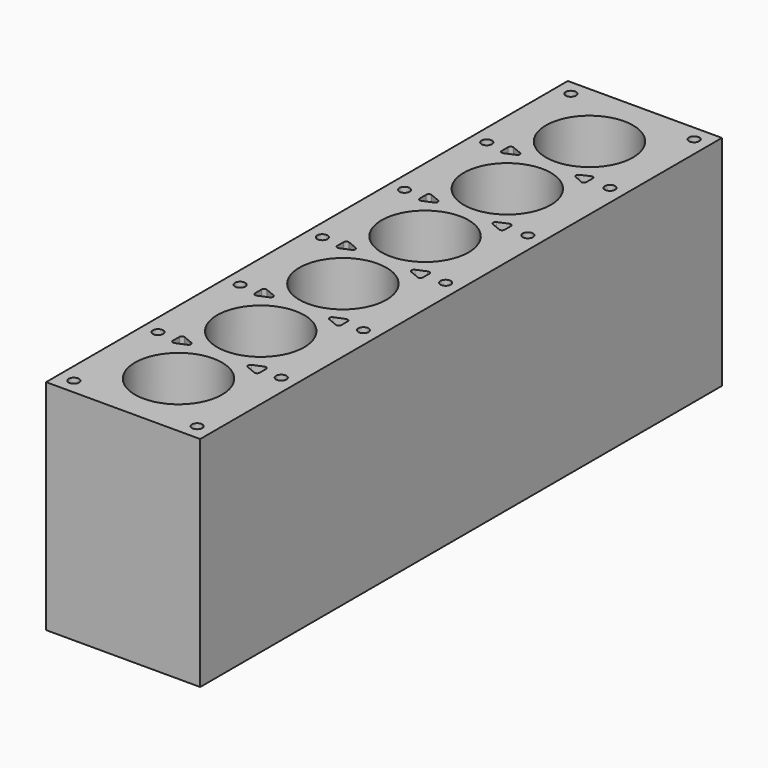
from build123d import *

# Parameters (mm, degrees)
F0_W     = 152.4
F0_H     = 644.906
F0_R     = 43.053
F1_DEPTH = 177.8
F3_D     = 10.16
F3_DEPTH = 50.8
F3_TIP   = 3.0523719447
F5_DEPTH = 101.6
F8_DEPTH = 38.1
F9_D     = 6.35
F9_DEPTH = 38.1
F9_TIP   = 1.9077324654
F10_R    = 6.35


# Not quite as in the source:
# - a feature names something its author has since deleted; it is built from what else it names


with BuildPart() as f1:
    # F0 (on Top) → F1 (new body)
    with BuildSketch(Plane.XY):
        with Locations((0, 22.9516405373)):
            Rectangle(F0_W, F0_H)
        with Locations((0, -231.0483594627)):
            Circle(F0_R, mode=Mode.SUBTRACT)
        with Locations((0, -129.4483594627)):
            Circle(F0_R, mode=Mode.SUBTRACT)
        with Locations((0, -27.8483594627)):
            Circle(F0_R, mode=Mode.SUBTRACT)
        with Locations((0, 73.7516405373)):
            Circle(F0_R, mode=Mode.SUBTRACT)
        with Locations((0, 175.3516405373)):
            Circle(F0_R, mode=Mode.SUBTRACT)
        with Locations((0, 276.9516405373)):
            Circle(F0_R, mode=Mode.SUBTRACT)
    extrude(amount=F1_DEPTH)

    # F3
    with Locations(Plane.XY.offset(177.8)):
        with Locations((-60.96, -284.2613594627), (60.96, -284.2613594627), (-60.96, -180.2483594627), (60.96, -180.2483594627), (-60.96, -78.6483594627), (60.96, -78.6483594627), (-60.96, 22.9516405373), (60.96, 22.9516405373), (-60.96, 124.5516405373), (60.96, 124.5516405373), (-60.96, 226.1516405373), (60.96, 226.1516405373), (-60.96, 330.1646405373), (60.96, 330.1646405373)):
            Hole(F3_D / 2, depth=F3_DEPTH)
            with Locations((0, 0, -(F3_DEPTH + F3_TIP / 2))):  # 118° drill point
                Cone(0, F3_D / 2, F3_TIP, mode=Mode.SUBTRACT)

    # F4 (on face) → F5 (cut)
    with BuildSketch(Plane.XY.offset(177.8)):
        with BuildLine():
            ThreePointArc((-39.5301250083, -173.9482047983), (-41.9112858201, -174.185525814), (-43.0385000083, -176.2963636216))
            Line((-43.0385000083, -176.2963636216), (-43.0385000083, -184.2003553039))
            ThreePointArc((-43.0385000083, -184.2003553039), (-41.9112858201, -186.3111931115), (-39.5301250083, -186.5485141272))
            Line((-39.5301250083, -186.5485141272), (-29.947149504, -182.596518286))
            ThreePointArc((-29.947149504, -182.596518286), (-28.375524504, -180.2483594627), (-29.947149504, -177.9002006395))
            Line((-29.947149504, -177.9002006395), (-39.5301250083, -173.9482047983))
        make_face()
        with BuildLine():
            Line((42.8050714591, -184.1785549312), (42.7631932188, -176.2809378323))
            ThreePointArc((42.7631932188, -176.2809378323), (41.6287769855, -174.1787422376), (39.2512218362, -173.9477486864))
            Line((39.2512218362, -173.9477486864), (29.7178532592, -177.8965572358))
            ThreePointArc((29.7178532592, -177.8965572358), (28.149861111, -180.2451799461), (29.7214853508, -182.5913737277))
            Line((29.7214853508, -182.5913737277), (39.2967321682, -186.5401822772))
            ThreePointArc((39.2967321682, -186.5401822772), (41.6834844647, -186.299108133), (42.8050714591, -184.1785549312))
        make_face()
        with BuildLine():
            ThreePointArc((-39.5301250083, -72.3482047983), (-41.9112858201, -72.585525814), (-43.0385000083, -74.6963636216))
            Line((-43.0385000083, -74.6963636216), (-43.0385000083, -82.6003553039))
            ThreePointArc((-43.0385000083, -82.6003553039), (-41.9112858201, -84.7111931115), (-39.5301250083, -84.9485141272))
            Line((-39.5301250083, -84.9485141272), (-29.947149504, -80.996518286))
            ThreePointArc((-29.947149504, -80.996518286), (-28.375524504, -78.6483594627), (-29.947149504, -76.3002006395))
            Line((-29.947149504, -76.3002006395), (-39.5301250083, -72.3482047983))
        make_face()
        with BuildLine():
            Line((42.2662900285, -82.5723412323), (42.2244772598, -74.6870711239))
            ThreePointArc((42.2244772598, -74.6870711239), (41.0880034509, -72.579426147), (38.7049289993, -72.3455539051))
            Line((38.7049289993, -72.3455539051), (29.1514032422, -76.2881889593))
            ThreePointArc((29.1514032422, -76.2881889593), (27.5756070282, -78.6451741517), (29.1550254915, -80.9997336057))
            Line((29.1550254915, -80.9997336057), (38.7503640173, -84.9423686599))
            ThreePointArc((38.7503640173, -84.9423686599), (41.1426684979, -84.6983979341), (42.2662900285, -82.5723412323))
        make_face()
        with BuildLine():
            ThreePointArc((-39.5301250083, 29.2517952017), (-41.9112858201, 29.014474186), (-43.0385000083, 26.9036363784))
            Line((-43.0385000083, 26.9036363784), (-43.0385000083, 18.9996446961))
            ThreePointArc((-43.0385000083, 18.9996446961), (-41.9112858201, 16.8888068885), (-39.5301250083, 16.6514858728))
            Line((-39.5301250083, 16.6514858728), (-29.947149504, 20.603481714))
            ThreePointArc((-29.947149504, 20.603481714), (-28.375524504, 22.9516405373), (-29.947149504, 25.2997993605))
            Line((-29.947149504, 25.2997993605), (-39.5301250083, 29.2517952017))
        make_face()
        with BuildLine():
            Line((41.7277221449, 18.9936006532), (41.6855505867, 26.946533154))
            ThreePointArc((41.6855505867, 26.946533154), (40.5605129606, 29.0230527195), (38.2087640486, 29.2396634781))
            Line((38.2087640486, 29.2396634781), (28.7869515979, 25.2631972277))
            ThreePointArc((28.7869515979, 25.2631972277), (27.2569622126, 22.9547929732), (28.7906370523, 20.6488356434))
            Line((28.7906370523, 20.6488356434), (38.2546210612, 16.672369393))
            ThreePointArc((38.2546210612, 16.672369393), (40.6154092138, 16.8989805748), (41.7277221449, 18.9936006532))
        make_face()
        with BuildLine():
            ThreePointArc((-39.2389715781, 130.8516052404), (-41.6215382557, 130.6118153154), (-42.7459306424, 128.4976098044))
            Line((-42.7459306424, 128.4976098044), (-42.7295716504, 120.5911560789))
            ThreePointArc((-42.7295716504, 120.5911560789), (-41.6001784129, 118.4841132501), (-39.2212020873, 118.2482526776))
            Line((-39.2212020873, 118.2482526776), (-29.635241547, 122.2014795403))
            ThreePointArc((-29.635241547, 122.2014795403), (-28.0636166616, 124.5504011364), (-29.6366520458, 126.8983783776))
            Line((-29.6366520458, 126.8983783776), (-39.2389715781, 130.8516052404))
        make_face()
        with BuildLine():
            Line((41.1269060209, 120.5623967021), (41.1269060209, 128.5408843724))
            ThreePointArc((41.1269060209, 128.5408843724), (40.0124074762, 130.6155991372), (37.6672454799, 130.8318480041))
            Line((37.6672454799, 130.8318480041), (28.2579874063, 126.8426041689))
            ThreePointArc((28.2579874063, 126.8426041689), (26.740926903, 124.5516405373), (28.2579874063, 122.2606769056))
            Line((28.2579874063, 122.2606769056), (37.6672454799, 118.2714330704))
            ThreePointArc((37.6672454799, 118.2714330704), (40.0124074762, 118.4876819373), (41.1269060209, 120.5623967021))
        make_face()
        with BuildLine():
            Line((-39.4786105583, 219.9656601087), (-29.866499751, 224.1805924273))
            ThreePointArc((-29.866499751, 224.1805924273), (-28.4228668084, 226.3396283374), (-29.8678000125, 228.4977942646))
            Line((-29.8678000125, 228.4977942646), (-39.5349560025, 232.4619589189))
            ThreePointArc((-39.5349560025, 232.4619589189), (-41.9134370658, 232.2213103618), (-43.0385000083, 230.1119698791))
            Line((-43.0385000083, 230.1119698791), (-43.0385000083, 222.2917467873))
            ThreePointArc((-43.0385000083, 222.2917467873), (-41.8879192273, 220.1655123145), (-39.4786105583, 219.9656601087))
        make_face()
        with BuildLine():
            Line((40.650672554, 222.1092328525), (40.6076142213, 230.2293979276))
            ThreePointArc((40.6076142213, 230.2293979276), (39.515765156, 232.1937343917), (37.2723493523, 232.3272920851))
            Line((37.2723493523, 232.3272920851), (28.7048957748, 228.2672095476))
            ThreePointArc((28.7048957748, 228.2672095476), (27.3697030623, 226.15467094), (28.7089851923, 224.0447225226))
            Line((28.7089851923, 224.0447225226), (37.3194971026, 219.9846399851))
            ThreePointArc((37.3194971026, 219.9846399851), (39.5711951198, 220.1279668388), (40.650672554, 222.1092328525))
        make_face()
    extrude(amount=-F5_DEPTH, mode=Mode.SUBTRACT)

    # F7 (on face) → F8 (join)
    with BuildSketch(Plane(origin=(0, 0, 0), x_dir=(1, 0, 0), z_dir=(0, 0, -1))):
        Polygon((76.2, -345.4046405373), (76.2, 299.4986176491), (76.2, 299.5013594627), (-76.2, 299.5013594627), (-76.2, -345.4046405373), align=None)
        Polygon((-60.96, -321.8358690433), (-60.96, 286.0599543583), (60.96, 286.0599543583), (60.96, -331.9680405373), (-60.96, -331.9680405373), align=None, mode=Mode.SUBTRACT)
    extrude(amount=F8_DEPTH)

    # F9 (one way)
    with BuildSketch(Plane.XY):
        with Locations((-68.58, -78.6483594627), (68.58, -78.6483594627)):
            Circle(F9_D / 2)
    extrude(amount=-F9_DEPTH, mode=Mode.SUBTRACT)
    with Locations(Plane.XY):
        with Locations((-68.58, -78.6483594627), (68.58, -78.6483594627)):
            with Locations((0, 0, -(F9_DEPTH + F9_TIP / 2))):  # 118° drill point
                Cone(0, F9_D / 2, F9_TIP, mode=Mode.SUBTRACT)

    # F10
    f10_edges = [f1.edges().sort_by_distance(p)[0] for p in [
        (60.96, -286.059954, -19.05),
        (-60.96, -286.059954, -19.05),
        (60.96, 331.968041, -19.05),
        (-60.96, 331.968041, -19.05),
    ]]
    fillet(f10_edges, radius=F10_R)


solid = f1.part
